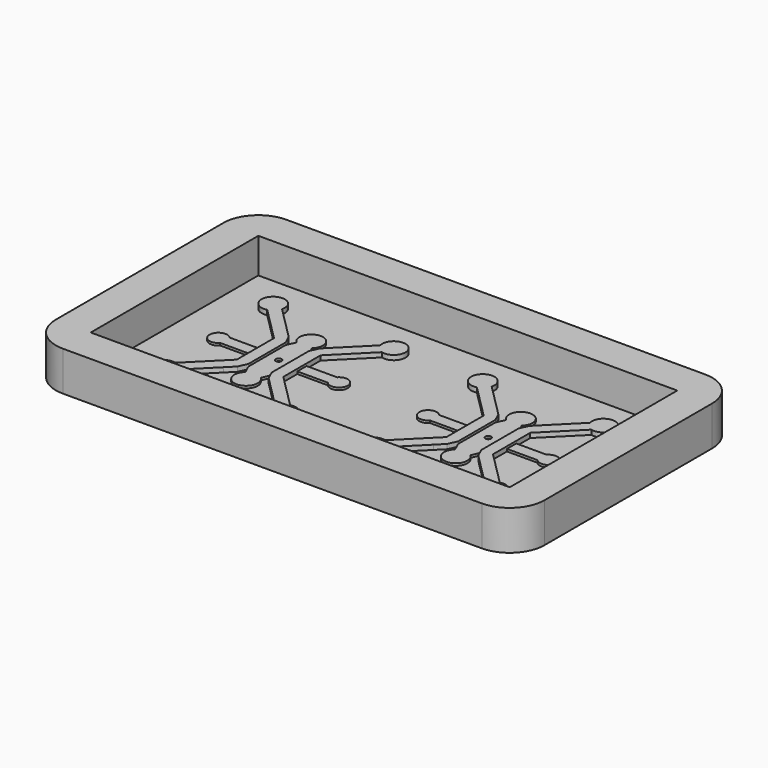
from build123d import *

# Parameters (mm, degrees)
F0_W     = 17.75
F0_H     = 18
F0_W_2   = 0.25
F1_DEPTH = 0.4
F2_DEPTH = 3
F3_DEPTH = 0.4
F4_DEPTH = 0.2


# Not quite as in the source:
# - a feature names something its author has since deleted; it is built from what else it names


with BuildPart() as f1:
    # F0 (on Top) → F1 (new body)
    with BuildSketch(Plane.XY):
        with BuildLine():
            Line((36, 21), (0, 21))
            ThreePointArc((0, 21), (-2.1213203436, 20.1213203436), (-3, 18))
            Line((-3, 18), (-3, 0))
            ThreePointArc((-3, 0), (-2.1213203436, -2.1213203436), (0, -3))
            Line((0, -3), (36, -3))
            ThreePointArc((36, -3), (38.1213203436, -2.1213203436), (39, 0))
            Line((39, 0), (39, 18))
            ThreePointArc((39, 18), (38.1213203436, 20.1213203436), (36, 21))
        make_face()
        Polygon((0, 0), (0, 18), (17.75, 18), (18, 18), (18.25, 18), (36, 18), (36, 0), (18.25, 0), (18, 0), (17.75, 0), align=None, mode=Mode.SUBTRACT)
        with Locations((8.875, 9)):
            Rectangle(F0_W, F0_H)
        with BuildLine():
            Line((9.6533412223, 11.6952957055), (9.9919033945, 10.9452957055))
            Line((9.9919033945, 10.9452957055), (10.3304655668, 11.6952957055))
            Line((10.3304655668, 11.6952957055), (10.9904227081, 12.3580254744))
            Line((10.9904227081, 12.3580254744), (13.2079580316, 14.5755632326))
            ThreePointArc((13.2079580316, 14.5755632326), (14.8809903029, 15.5414897832), (13.9150646707, 13.8684569817))
            Line((13.9150646707, 13.8684569817), (10.9919033945, 10.9452957055))
            Line((10.9919033945, 10.9452957055), (10.9919033945, 9.4452957055))
            Line((10.9919033945, 9.4452957055), (13.6148667214, 9.4452957055))
            ThreePointArc((13.6148667214, 9.4452957055), (13.70376764, 9.5296679116), (13.8052234095, 9.5984339593))
            ThreePointArc((13.8052234095, 9.5984339593), (14.9138690208, 8.823141097), (13.6148667214, 8.4452957055))
            Line((13.6148667214, 8.4452957055), (10.9919033945, 8.4452957055))
            Line((10.9919033945, 8.4452957055), (10.9919033945, 6.9452957055))
            Line((10.9919033945, 6.9452957055), (13.9150646707, 4.0221344294))
            ThreePointArc((13.9150646707, 4.0221344294), (14.8809903029, 2.3491016278), (13.2079580316, 3.3150281785))
            Line((13.2079580316, 3.3150281785), (10.9904227081, 5.5325659367))
            Line((10.9904227081, 5.5325659367), (10.3304655668, 6.1952957055))
            Line((10.3304655668, 6.1952957055), (9.9919033945, 6.9452957055))
            Line((9.9919033945, 6.9452957055), (9.6533412223, 6.1952957055))
            ThreePointArc((9.6533412223, 6.1952957055), (8.9919033945, 4.4452957055), (8.3304655668, 6.1952957055))
            Line((8.3304655668, 6.1952957055), (7.9919033945, 6.9452957055))
            Line((7.9919033945, 6.9452957055), (7.6533412223, 6.1952957055))
            Line((7.6533412223, 6.1952957055), (6.993384081, 5.5325659367))
            Line((6.993384081, 5.5325659367), (4.7758487575, 3.3150281785))
            ThreePointArc((4.7758487575, 3.3150281785), (3.1028164862, 2.3491016278), (4.0687421184, 4.0221344294))
            Line((4.0687421184, 4.0221344294), (6.9919033945, 6.9452957055))
            Line((6.9919033945, 6.9452957055), (6.9919033945, 8.4452957055))
            Line((6.9919033945, 8.4452957055), (4.3689400677, 8.4452957055))
            ThreePointArc((4.3689400677, 8.4452957055), (3.0699377683, 8.823141097), (4.1785833795, 9.5984339593))
            ThreePointArc((4.1785833795, 9.5984339593), (4.2800391491, 9.5296679116), (4.3689400677, 9.4452957055))
            Line((4.3689400677, 9.4452957055), (6.9919033945, 9.4452957055))
            Line((6.9919033945, 9.4452957055), (6.9919033945, 10.9452957055))
            Line((6.9919033945, 10.9452957055), (4.0687421184, 13.8684569817))
            ThreePointArc((4.0687421184, 13.8684569817), (3.1028164862, 15.5414897832), (4.7758487575, 14.5755632326))
            Line((4.7758487575, 14.5755632326), (6.993384081, 12.3580254744))
            Line((6.993384081, 12.3580254744), (7.6533412223, 11.6952957055))
            Line((7.6533412223, 11.6952957055), (7.9919033945, 10.9452957055))
            Line((7.9919033945, 10.9452957055), (8.3304655668, 11.6952957055))
            ThreePointArc((8.3304655668, 11.6952957055), (8.9919033945, 13.4452957055), (9.6533412223, 11.6952957055))
        make_face(mode=Mode.SUBTRACT)
        with Locations((27.125, 9)):
            Rectangle(F0_W, F0_H)
        with BuildLine():
            Line((27.6695344332, 11.6952957055), (28.0080966055, 10.9452957055))
            Line((28.0080966055, 10.9452957055), (28.3466587777, 11.6952957055))
            Line((28.3466587777, 11.6952957055), (29.006615919, 12.3580254744))
            Line((29.006615919, 12.3580254744), (31.2241512425, 14.5755632326))
            ThreePointArc((31.2241512425, 14.5755632326), (32.8971835138, 15.5414897832), (31.9312578816, 13.8684569817))
            Line((31.9312578816, 13.8684569817), (29.0080966055, 10.9452957055))
            Line((29.0080966055, 10.9452957055), (29.0080966055, 9.4452957055))
            Line((29.0080966055, 9.4452957055), (31.6310599323, 9.4452957055))
            ThreePointArc((31.6310599323, 9.4452957055), (31.7199608509, 9.5296679116), (31.8214166205, 9.5984339593))
            ThreePointArc((31.8214166205, 9.5984339593), (32.9300622317, 8.823141097), (31.6310599323, 8.4452957055))
            Line((31.6310599323, 8.4452957055), (29.0080966055, 8.4452957055))
            Line((29.0080966055, 8.4452957055), (29.0080966055, 6.9452957055))
            Line((29.0080966055, 6.9452957055), (31.9312578816, 4.0221344294))
            ThreePointArc((31.9312578816, 4.0221344294), (32.8971835138, 2.3491016278), (31.2241512425, 3.3150281785))
            Line((31.2241512425, 3.3150281785), (29.006615919, 5.5325659367))
            Line((29.006615919, 5.5325659367), (28.3466587777, 6.1952957055))
            Line((28.3466587777, 6.1952957055), (28.0080966055, 6.9452957055))
            Line((28.0080966055, 6.9452957055), (27.6695344332, 6.1952957055))
            ThreePointArc((27.6695344332, 6.1952957055), (27.0080966055, 4.4452957055), (26.3466587777, 6.1952957055))
            Line((26.3466587777, 6.1952957055), (26.0080966055, 6.9452957055))
            Line((26.0080966055, 6.9452957055), (25.6695344332, 6.1952957055))
            Line((25.6695344332, 6.1952957055), (25.0095772919, 5.5325659367))
            Line((25.0095772919, 5.5325659367), (22.7920419684, 3.3150281785))
            ThreePointArc((22.7920419684, 3.3150281785), (21.1190096971, 2.3491016278), (22.0849353293, 4.0221344294))
            Line((22.0849353293, 4.0221344294), (25.0080966055, 6.9452957055))
            Line((25.0080966055, 6.9452957055), (25.0080966055, 8.4452957055))
            Line((25.0080966055, 8.4452957055), (22.3851332786, 8.4452957055))
            ThreePointArc((22.3851332786, 8.4452957055), (21.0861309792, 8.823141097), (22.1947765905, 9.5984339593))
            ThreePointArc((22.1947765905, 9.5984339593), (22.29623236, 9.5296679116), (22.3851332786, 9.4452957055))
            Line((22.3851332786, 9.4452957055), (25.0080966055, 9.4452957055))
            Line((25.0080966055, 9.4452957055), (25.0080966055, 10.9452957055))
            Line((25.0080966055, 10.9452957055), (22.0849353293, 13.8684569817))
            ThreePointArc((22.0849353293, 13.8684569817), (21.1190096971, 15.5414897832), (22.7920419684, 14.5755632326))
            Line((22.7920419684, 14.5755632326), (25.0095772919, 12.3580254744))
            Line((25.0095772919, 12.3580254744), (25.6695344332, 11.6952957055))
            Line((25.6695344332, 11.6952957055), (26.0080966055, 10.9452957055))
            Line((26.0080966055, 10.9452957055), (26.3466587777, 11.6952957055))
            ThreePointArc((26.3466587777, 11.6952957055), (27.0080966055, 13.4452957055), (27.6695344332, 11.6952957055))
        make_face(mode=Mode.SUBTRACT)
        with BuildLine():
            Line((26.0080966055, 8.9452957055), (26.0080966055, 10.9452957055))
            Line((26.0080966055, 10.9452957055), (25.6695344332, 11.6952957055))
            Line((25.6695344332, 11.6952957055), (25.0095772919, 12.3580254744))
            Line((25.0095772919, 12.3580254744), (22.7920419684, 14.5755632326))
            ThreePointArc((22.7920419684, 14.5755632326), (21.1190096971, 15.5414897832), (22.0849353293, 13.8684569817))
            Line((22.0849353293, 13.8684569817), (25.0080966055, 10.9452957055))
            Line((25.0080966055, 10.9452957055), (25.0080966055, 9.4452957055))
            Line((25.0080966055, 9.4452957055), (25.0080966055, 8.9452957055))
            Line((25.0080966055, 8.9452957055), (25.0080966055, 8.4452957055))
            Line((25.0080966055, 8.4452957055), (25.0080966055, 6.9452957055))
            Line((25.0080966055, 6.9452957055), (22.0849353293, 4.0221344294))
            ThreePointArc((22.0849353293, 4.0221344294), (21.1190096971, 2.3491016278), (22.7920419684, 3.3150281785))
            Line((22.7920419684, 3.3150281785), (25.0095772919, 5.5325659367))
            Line((25.0095772919, 5.5325659367), (25.6695344332, 6.1952957055))
            Line((25.6695344332, 6.1952957055), (26.0080966055, 6.9452957055))
            Line((26.0080966055, 6.9452957055), (26.0080966055, 8.9452957055))
        make_face()
        with BuildLine():
            Line((28.3466587777, 11.6952957055), (28.0080966055, 10.9452957055))
            Line((28.0080966055, 10.9452957055), (28.0080966055, 8.9452957055))
            Line((28.0080966055, 8.9452957055), (28.0080966055, 6.9452957055))
            Line((28.0080966055, 6.9452957055), (28.3466587777, 6.1952957055))
            Line((28.3466587777, 6.1952957055), (29.006615919, 5.5325659367))
            Line((29.006615919, 5.5325659367), (31.2241512425, 3.3150281785))
            ThreePointArc((31.2241512425, 3.3150281785), (32.8971835138, 2.3491016278), (31.9312578816, 4.0221344294))
            Line((31.9312578816, 4.0221344294), (29.0080966055, 6.9452957055))
            Line((29.0080966055, 6.9452957055), (29.0080966055, 8.4452957055))
            Line((29.0080966055, 8.4452957055), (29.0080966055, 8.9452957055))
            Line((29.0080966055, 8.9452957055), (29.0080966055, 9.4452957055))
            Line((29.0080966055, 9.4452957055), (29.0080966055, 10.9452957055))
            Line((29.0080966055, 10.9452957055), (31.9312578816, 13.8684569817))
            ThreePointArc((31.9312578816, 13.8684569817), (32.8971835138, 15.5414897832), (31.2241512425, 14.5755632326))
            Line((31.2241512425, 14.5755632326), (29.006615919, 12.3580254744))
            Line((29.006615919, 12.3580254744), (28.3466587777, 11.6952957055))
        make_face()
        with BuildLine():
            Line((7.9919033945, 8.9452957055), (7.9919033945, 10.9452957055))
            Line((7.9919033945, 10.9452957055), (7.6533412223, 11.6952957055))
            Line((7.6533412223, 11.6952957055), (6.993384081, 12.3580254744))
            Line((6.993384081, 12.3580254744), (4.7758487575, 14.5755632326))
            ThreePointArc((4.7758487575, 14.5755632326), (3.1028164862, 15.5414897832), (4.0687421184, 13.8684569817))
            Line((4.0687421184, 13.8684569817), (6.9919033945, 10.9452957055))
            Line((6.9919033945, 10.9452957055), (6.9919033945, 9.4452957055))
            Line((6.9919033945, 9.4452957055), (6.9919033945, 8.9452957055))
            Line((6.9919033945, 8.9452957055), (6.9919033945, 8.4452957055))
            Line((6.9919033945, 8.4452957055), (6.9919033945, 6.9452957055))
            Line((6.9919033945, 6.9452957055), (4.0687421184, 4.0221344294))
            ThreePointArc((4.0687421184, 4.0221344294), (3.1028164862, 2.3491016278), (4.7758487575, 3.3150281785))
            Line((4.7758487575, 3.3150281785), (6.993384081, 5.5325659367))
            Line((6.993384081, 5.5325659367), (7.6533412223, 6.1952957055))
            Line((7.6533412223, 6.1952957055), (7.9919033945, 6.9452957055))
            Line((7.9919033945, 6.9452957055), (7.9919033945, 8.9452957055))
        make_face()
        with BuildLine():
            Line((9.9919033945, 10.9452957055), (9.9919033945, 8.9452957055))
            Line((9.9919033945, 8.9452957055), (9.9919033945, 6.9452957055))
            Line((9.9919033945, 6.9452957055), (10.3304655668, 6.1952957055))
            Line((10.3304655668, 6.1952957055), (10.9904227081, 5.5325659367))
            Line((10.9904227081, 5.5325659367), (13.2079580316, 3.3150281785))
            ThreePointArc((13.2079580316, 3.3150281785), (14.8809903029, 2.3491016278), (13.9150646707, 4.0221344294))
            Line((13.9150646707, 4.0221344294), (10.9919033945, 6.9452957055))
            Line((10.9919033945, 6.9452957055), (10.9919033945, 8.4452957055))
            Line((10.9919033945, 8.4452957055), (10.9919033945, 8.9452957055))
            Line((10.9919033945, 8.9452957055), (10.9919033945, 9.4452957055))
            Line((10.9919033945, 9.4452957055), (10.9919033945, 10.9452957055))
            Line((10.9919033945, 10.9452957055), (13.9150646707, 13.8684569817))
            ThreePointArc((13.9150646707, 13.8684569817), (14.8809903029, 15.5414897832), (13.2079580316, 14.5755632326))
            Line((13.2079580316, 14.5755632326), (10.9904227081, 12.3580254744))
            Line((10.9904227081, 12.3580254744), (10.3304655668, 11.6952957055))
            Line((10.3304655668, 11.6952957055), (9.9919033945, 10.9452957055))
        make_face()
        with BuildLine():
            Line((28.0080966055, 8.9452957055), (28.0080966055, 10.9452957055))
            Line((28.0080966055, 10.9452957055), (27.6695344332, 11.6952957055))
            ThreePointArc((27.6695344332, 11.6952957055), (27.0080966055, 13.4452957055), (26.3466587777, 11.6952957055))
            Line((26.3466587777, 11.6952957055), (26.0080966055, 10.9452957055))
            Line((26.0080966055, 10.9452957055), (26.0080966055, 8.9452957055))
            Line((26.0080966055, 8.9452957055), (26.0080966055, 6.9452957055))
            Line((26.0080966055, 6.9452957055), (26.3466587777, 6.1952957055))
            ThreePointArc((26.3466587777, 6.1952957055), (27.0080966055, 4.4452957055), (27.6695344332, 6.1952957055))
            Line((27.6695344332, 6.1952957055), (28.0080966055, 6.9452957055))
            Line((28.0080966055, 6.9452957055), (28.0080966055, 8.9452957055))
        make_face()
        with BuildLine():
            ThreePointArc((27.0080966055, 9.1952957055), (27.1848733008, 9.1220724008), (27.2580966055, 8.9452957055))
            ThreePointArc((27.2580966055, 8.9452957055), (27.1848733008, 8.7685190102), (27.0080966055, 8.6952957055))
            ThreePointArc((27.0080966055, 8.6952957055), (26.7580966055, 8.9452957055), (27.0080966055, 9.1952957055))
        make_face(mode=Mode.SUBTRACT)
        with BuildLine():
            Line((9.9919033945, 6.9452957055), (9.9919033945, 8.9452957055))
            Line((9.9919033945, 8.9452957055), (9.9919033945, 10.9452957055))
            Line((9.9919033945, 10.9452957055), (9.6533412223, 11.6952957055))
            ThreePointArc((9.6533412223, 11.6952957055), (8.9919033945, 13.4452957055), (8.3304655668, 11.6952957055))
            Line((8.3304655668, 11.6952957055), (7.9919033945, 10.9452957055))
            Line((7.9919033945, 10.9452957055), (7.9919033945, 8.9452957055))
            Line((7.9919033945, 8.9452957055), (7.9919033945, 6.9452957055))
            Line((7.9919033945, 6.9452957055), (8.3304655668, 6.1952957055))
            ThreePointArc((8.3304655668, 6.1952957055), (8.9919033945, 4.4452957055), (9.6533412223, 6.1952957055))
            Line((9.6533412223, 6.1952957055), (9.9919033945, 6.9452957055))
        make_face()
        with BuildLine():
            ThreePointArc((8.9919033945, 9.1952957055), (9.1686800898, 9.1220724008), (9.2419033945, 8.9452957055))
            ThreePointArc((9.2419033945, 8.9452957055), (9.1686800898, 8.7685190102), (8.9919033945, 8.6952957055))
            ThreePointArc((8.9919033945, 8.6952957055), (8.7419033945, 8.9452957055), (8.9919033945, 9.1952957055))
        make_face(mode=Mode.SUBTRACT)
        with Locations((17.875, 9)):
            Rectangle(F0_W_2, F0_H)
        with Locations((18.125, 9)):
            Rectangle(F0_W_2, F0_H)
        with BuildLine():
            Line((6.9919033945, 8.9452957055), (6.9919033945, 9.4452957055))
            Line((6.9919033945, 9.4452957055), (4.3689400677, 9.4452957055))
            ThreePointArc((4.3689400677, 9.4452957055), (4.2800391491, 9.5296679116), (4.1785833795, 9.5984339593))
            ThreePointArc((4.1785833795, 9.5984339593), (3.0699377683, 8.823141097), (4.3689400677, 8.4452957055))
            Line((4.3689400677, 8.4452957055), (6.9919033945, 8.4452957055))
            Line((6.9919033945, 8.4452957055), (6.9919033945, 8.9452957055))
        make_face()
        with BuildLine():
            Line((31.6310599323, 9.4452957055), (29.0080966055, 9.4452957055))
            Line((29.0080966055, 9.4452957055), (29.0080966055, 8.9452957055))
            Line((29.0080966055, 8.9452957055), (29.0080966055, 8.4452957055))
            Line((29.0080966055, 8.4452957055), (31.6310599323, 8.4452957055))
            ThreePointArc((31.6310599323, 8.4452957055), (32.9300622317, 8.823141097), (31.8214166205, 9.5984339593))
            ThreePointArc((31.8214166205, 9.5984339593), (31.7199608509, 9.5296679116), (31.6310599323, 9.4452957055))
        make_face()
        with BuildLine():
            Line((25.0080966055, 8.9452957055), (25.0080966055, 9.4452957055))
            Line((25.0080966055, 9.4452957055), (22.3851332786, 9.4452957055))
            ThreePointArc((22.3851332786, 9.4452957055), (22.29623236, 9.5296679116), (22.1947765905, 9.5984339593))
            ThreePointArc((22.1947765905, 9.5984339593), (21.0861309792, 8.823141097), (22.3851332786, 8.4452957055))
            Line((22.3851332786, 8.4452957055), (25.0080966055, 8.4452957055))
            Line((25.0080966055, 8.4452957055), (25.0080966055, 8.9452957055))
        make_face()
        with BuildLine():
            Line((13.6148667214, 9.4452957055), (10.9919033945, 9.4452957055))
            Line((10.9919033945, 9.4452957055), (10.9919033945, 8.9452957055))
            Line((10.9919033945, 8.9452957055), (10.9919033945, 8.4452957055))
            Line((10.9919033945, 8.4452957055), (13.6148667214, 8.4452957055))
            ThreePointArc((13.6148667214, 8.4452957055), (14.9138690208, 8.823141097), (13.8052234095, 9.5984339593))
            ThreePointArc((13.8052234095, 9.5984339593), (13.70376764, 9.5296679116), (13.6148667214, 9.4452957055))
        make_face()
        with BuildLine():
            ThreePointArc((8.9919033945, 8.6952957055), (9.1686800898, 8.7685190102), (9.2419033945, 8.9452957055))
            ThreePointArc((9.2419033945, 8.9452957055), (9.1686800898, 9.1220724008), (8.9919033945, 9.1952957055))
            Line((8.9919033945, 9.1952957055), (8.9919033945, 8.6952957055))
        make_face()
        with BuildLine():
            ThreePointArc((27.0080966055, 8.6952957055), (27.1848733008, 8.7685190102), (27.2580966055, 8.9452957055))
            ThreePointArc((27.2580966055, 8.9452957055), (27.1848733008, 9.1220724008), (27.0080966055, 9.1952957055))
            Line((27.0080966055, 9.1952957055), (27.0080966055, 8.6952957055))
        make_face()
        with BuildLine():
            Line((8.9919033945, 8.6952957055), (8.9919033945, 9.1952957055))
            ThreePointArc((8.9919033945, 9.1952957055), (8.7419033945, 8.9452957055), (8.9919033945, 8.6952957055))
        make_face()
        with BuildLine():
            Line((27.0080966055, 8.6952957055), (27.0080966055, 9.1952957055))
            ThreePointArc((27.0080966055, 9.1952957055), (26.7580966055, 8.9452957055), (27.0080966055, 8.6952957055))
        make_face()
    extrude(amount=-F1_DEPTH)

    # F0 (on Top) → F2 (join)
    with BuildSketch(Plane.XY):
        with BuildLine():
            Line((36, 21), (0, 21))
            ThreePointArc((0, 21), (-2.1213203436, 20.1213203436), (-3, 18))
            Line((-3, 18), (-3, 0))
            ThreePointArc((-3, 0), (-2.1213203436, -2.1213203436), (0, -3))
            Line((0, -3), (36, -3))
            ThreePointArc((36, -3), (38.1213203436, -2.1213203436), (39, 0))
            Line((39, 0), (39, 18))
            ThreePointArc((39, 18), (38.1213203436, 20.1213203436), (36, 21))
        make_face()
        Polygon((0, 0), (0, 18), (17.75, 18), (18, 18), (18.25, 18), (36, 18), (36, 0), (18.25, 0), (18, 0), (17.75, 0), align=None, mode=Mode.SUBTRACT)
    extrude(amount=F2_DEPTH)

    # F0 (on Top) → F3 (join)
    with BuildSketch(Plane.XY):
        with BuildLine():
            Line((7.9919033945, 8.9452957055), (7.9919033945, 10.9452957055))
            Line((7.9919033945, 10.9452957055), (7.6533412223, 11.6952957055))
            Line((7.6533412223, 11.6952957055), (6.993384081, 12.3580254744))
            Line((6.993384081, 12.3580254744), (4.7758487575, 14.5755632326))
            ThreePointArc((4.7758487575, 14.5755632326), (3.1028164862, 15.5414897832), (4.0687421184, 13.8684569817))
            Line((4.0687421184, 13.8684569817), (6.9919033945, 10.9452957055))
            Line((6.9919033945, 10.9452957055), (6.9919033945, 9.4452957055))
            Line((6.9919033945, 9.4452957055), (6.9919033945, 8.9452957055))
            Line((6.9919033945, 8.9452957055), (6.9919033945, 8.4452957055))
            Line((6.9919033945, 8.4452957055), (6.9919033945, 6.9452957055))
            Line((6.9919033945, 6.9452957055), (4.0687421184, 4.0221344294))
            ThreePointArc((4.0687421184, 4.0221344294), (3.1028164862, 2.3491016278), (4.7758487575, 3.3150281785))
            Line((4.7758487575, 3.3150281785), (6.993384081, 5.5325659367))
            Line((6.993384081, 5.5325659367), (7.6533412223, 6.1952957055))
            Line((7.6533412223, 6.1952957055), (7.9919033945, 6.9452957055))
            Line((7.9919033945, 6.9452957055), (7.9919033945, 8.9452957055))
        make_face()
        with BuildLine():
            Line((9.9919033945, 10.9452957055), (9.9919033945, 8.9452957055))
            Line((9.9919033945, 8.9452957055), (9.9919033945, 6.9452957055))
            Line((9.9919033945, 6.9452957055), (10.3304655668, 6.1952957055))
            Line((10.3304655668, 6.1952957055), (10.9904227081, 5.5325659367))
            Line((10.9904227081, 5.5325659367), (13.2079580316, 3.3150281785))
            ThreePointArc((13.2079580316, 3.3150281785), (14.8809903029, 2.3491016278), (13.9150646707, 4.0221344294))
            Line((13.9150646707, 4.0221344294), (10.9919033945, 6.9452957055))
            Line((10.9919033945, 6.9452957055), (10.9919033945, 8.4452957055))
            Line((10.9919033945, 8.4452957055), (10.9919033945, 8.9452957055))
            Line((10.9919033945, 8.9452957055), (10.9919033945, 9.4452957055))
            Line((10.9919033945, 9.4452957055), (10.9919033945, 10.9452957055))
            Line((10.9919033945, 10.9452957055), (13.9150646707, 13.8684569817))
            ThreePointArc((13.9150646707, 13.8684569817), (14.8809903029, 15.5414897832), (13.2079580316, 14.5755632326))
            Line((13.2079580316, 14.5755632326), (10.9904227081, 12.3580254744))
            Line((10.9904227081, 12.3580254744), (10.3304655668, 11.6952957055))
            Line((10.3304655668, 11.6952957055), (9.9919033945, 10.9452957055))
        make_face()
        with BuildLine():
            Line((26.0080966055, 8.9452957055), (26.0080966055, 10.9452957055))
            Line((26.0080966055, 10.9452957055), (25.6695344332, 11.6952957055))
            Line((25.6695344332, 11.6952957055), (25.0095772919, 12.3580254744))
            Line((25.0095772919, 12.3580254744), (22.7920419684, 14.5755632326))
            ThreePointArc((22.7920419684, 14.5755632326), (21.1190096971, 15.5414897832), (22.0849353293, 13.8684569817))
            Line((22.0849353293, 13.8684569817), (25.0080966055, 10.9452957055))
            Line((25.0080966055, 10.9452957055), (25.0080966055, 9.4452957055))
            Line((25.0080966055, 9.4452957055), (25.0080966055, 8.9452957055))
            Line((25.0080966055, 8.9452957055), (25.0080966055, 8.4452957055))
            Line((25.0080966055, 8.4452957055), (25.0080966055, 6.9452957055))
            Line((25.0080966055, 6.9452957055), (22.0849353293, 4.0221344294))
            ThreePointArc((22.0849353293, 4.0221344294), (21.1190096971, 2.3491016278), (22.7920419684, 3.3150281785))
            Line((22.7920419684, 3.3150281785), (25.0095772919, 5.5325659367))
            Line((25.0095772919, 5.5325659367), (25.6695344332, 6.1952957055))
            Line((25.6695344332, 6.1952957055), (26.0080966055, 6.9452957055))
            Line((26.0080966055, 6.9452957055), (26.0080966055, 8.9452957055))
        make_face()
        with BuildLine():
            Line((28.3466587777, 11.6952957055), (28.0080966055, 10.9452957055))
            Line((28.0080966055, 10.9452957055), (28.0080966055, 8.9452957055))
            Line((28.0080966055, 8.9452957055), (28.0080966055, 6.9452957055))
            Line((28.0080966055, 6.9452957055), (28.3466587777, 6.1952957055))
            Line((28.3466587777, 6.1952957055), (29.006615919, 5.5325659367))
            Line((29.006615919, 5.5325659367), (31.2241512425, 3.3150281785))
            ThreePointArc((31.2241512425, 3.3150281785), (32.8971835138, 2.3491016278), (31.9312578816, 4.0221344294))
            Line((31.9312578816, 4.0221344294), (29.0080966055, 6.9452957055))
            Line((29.0080966055, 6.9452957055), (29.0080966055, 8.4452957055))
            Line((29.0080966055, 8.4452957055), (29.0080966055, 8.9452957055))
            Line((29.0080966055, 8.9452957055), (29.0080966055, 9.4452957055))
            Line((29.0080966055, 9.4452957055), (29.0080966055, 10.9452957055))
            Line((29.0080966055, 10.9452957055), (31.9312578816, 13.8684569817))
            ThreePointArc((31.9312578816, 13.8684569817), (32.8971835138, 15.5414897832), (31.2241512425, 14.5755632326))
            Line((31.2241512425, 14.5755632326), (29.006615919, 12.3580254744))
            Line((29.006615919, 12.3580254744), (28.3466587777, 11.6952957055))
        make_face()
    extrude(amount=F3_DEPTH)

    # F0 (on Top) → F4 (join)
    with BuildSketch(Plane.XY):
        with BuildLine():
            Line((6.9919033945, 8.9452957055), (6.9919033945, 9.4452957055))
            Line((6.9919033945, 9.4452957055), (4.3689400677, 9.4452957055))
            ThreePointArc((4.3689400677, 9.4452957055), (4.2800391491, 9.5296679116), (4.1785833795, 9.5984339593))
            ThreePointArc((4.1785833795, 9.5984339593), (3.0699377683, 8.823141097), (4.3689400677, 8.4452957055))
            Line((4.3689400677, 8.4452957055), (6.9919033945, 8.4452957055))
            Line((6.9919033945, 8.4452957055), (6.9919033945, 8.9452957055))
        make_face()
        with BuildLine():
            Line((9.9919033945, 6.9452957055), (9.9919033945, 8.9452957055))
            Line((9.9919033945, 8.9452957055), (9.9919033945, 10.9452957055))
            Line((9.9919033945, 10.9452957055), (9.6533412223, 11.6952957055))
            ThreePointArc((9.6533412223, 11.6952957055), (8.9919033945, 13.4452957055), (8.3304655668, 11.6952957055))
            Line((8.3304655668, 11.6952957055), (7.9919033945, 10.9452957055))
            Line((7.9919033945, 10.9452957055), (7.9919033945, 8.9452957055))
            Line((7.9919033945, 8.9452957055), (7.9919033945, 6.9452957055))
            Line((7.9919033945, 6.9452957055), (8.3304655668, 6.1952957055))
            ThreePointArc((8.3304655668, 6.1952957055), (8.9919033945, 4.4452957055), (9.6533412223, 6.1952957055))
            Line((9.6533412223, 6.1952957055), (9.9919033945, 6.9452957055))
        make_face()
        with BuildLine():
            ThreePointArc((8.9919033945, 9.1952957055), (9.1686800898, 9.1220724008), (9.2419033945, 8.9452957055))
            ThreePointArc((9.2419033945, 8.9452957055), (9.1686800898, 8.7685190102), (8.9919033945, 8.6952957055))
            ThreePointArc((8.9919033945, 8.6952957055), (8.7419033945, 8.9452957055), (8.9919033945, 9.1952957055))
        make_face(mode=Mode.SUBTRACT)
        with BuildLine():
            Line((13.6148667214, 9.4452957055), (10.9919033945, 9.4452957055))
            Line((10.9919033945, 9.4452957055), (10.9919033945, 8.9452957055))
            Line((10.9919033945, 8.9452957055), (10.9919033945, 8.4452957055))
            Line((10.9919033945, 8.4452957055), (13.6148667214, 8.4452957055))
            ThreePointArc((13.6148667214, 8.4452957055), (14.9138690208, 8.823141097), (13.8052234095, 9.5984339593))
            ThreePointArc((13.8052234095, 9.5984339593), (13.70376764, 9.5296679116), (13.6148667214, 9.4452957055))
        make_face()
        with BuildLine():
            Line((25.0080966055, 8.9452957055), (25.0080966055, 9.4452957055))
            Line((25.0080966055, 9.4452957055), (22.3851332786, 9.4452957055))
            ThreePointArc((22.3851332786, 9.4452957055), (22.29623236, 9.5296679116), (22.1947765905, 9.5984339593))
            ThreePointArc((22.1947765905, 9.5984339593), (21.0861309792, 8.823141097), (22.3851332786, 8.4452957055))
            Line((22.3851332786, 8.4452957055), (25.0080966055, 8.4452957055))
            Line((25.0080966055, 8.4452957055), (25.0080966055, 8.9452957055))
        make_face()
        with BuildLine():
            Line((28.0080966055, 8.9452957055), (28.0080966055, 10.9452957055))
            Line((28.0080966055, 10.9452957055), (27.6695344332, 11.6952957055))
            ThreePointArc((27.6695344332, 11.6952957055), (27.0080966055, 13.4452957055), (26.3466587777, 11.6952957055))
            Line((26.3466587777, 11.6952957055), (26.0080966055, 10.9452957055))
            Line((26.0080966055, 10.9452957055), (26.0080966055, 8.9452957055))
            Line((26.0080966055, 8.9452957055), (26.0080966055, 6.9452957055))
            Line((26.0080966055, 6.9452957055), (26.3466587777, 6.1952957055))
            ThreePointArc((26.3466587777, 6.1952957055), (27.0080966055, 4.4452957055), (27.6695344332, 6.1952957055))
            Line((27.6695344332, 6.1952957055), (28.0080966055, 6.9452957055))
            Line((28.0080966055, 6.9452957055), (28.0080966055, 8.9452957055))
        make_face()
        with BuildLine():
            ThreePointArc((27.0080966055, 9.1952957055), (27.1848733008, 9.1220724008), (27.2580966055, 8.9452957055))
            ThreePointArc((27.2580966055, 8.9452957055), (27.1848733008, 8.7685190102), (27.0080966055, 8.6952957055))
            ThreePointArc((27.0080966055, 8.6952957055), (26.7580966055, 8.9452957055), (27.0080966055, 9.1952957055))
        make_face(mode=Mode.SUBTRACT)
        with BuildLine():
            Line((31.6310599323, 9.4452957055), (29.0080966055, 9.4452957055))
            Line((29.0080966055, 9.4452957055), (29.0080966055, 8.9452957055))
            Line((29.0080966055, 8.9452957055), (29.0080966055, 8.4452957055))
            Line((29.0080966055, 8.4452957055), (31.6310599323, 8.4452957055))
            ThreePointArc((31.6310599323, 8.4452957055), (32.9300622317, 8.823141097), (31.8214166205, 9.5984339593))
            ThreePointArc((31.8214166205, 9.5984339593), (31.7199608509, 9.5296679116), (31.6310599323, 9.4452957055))
        make_face()
    extrude(amount=F4_DEPTH)


solid = f1.part
